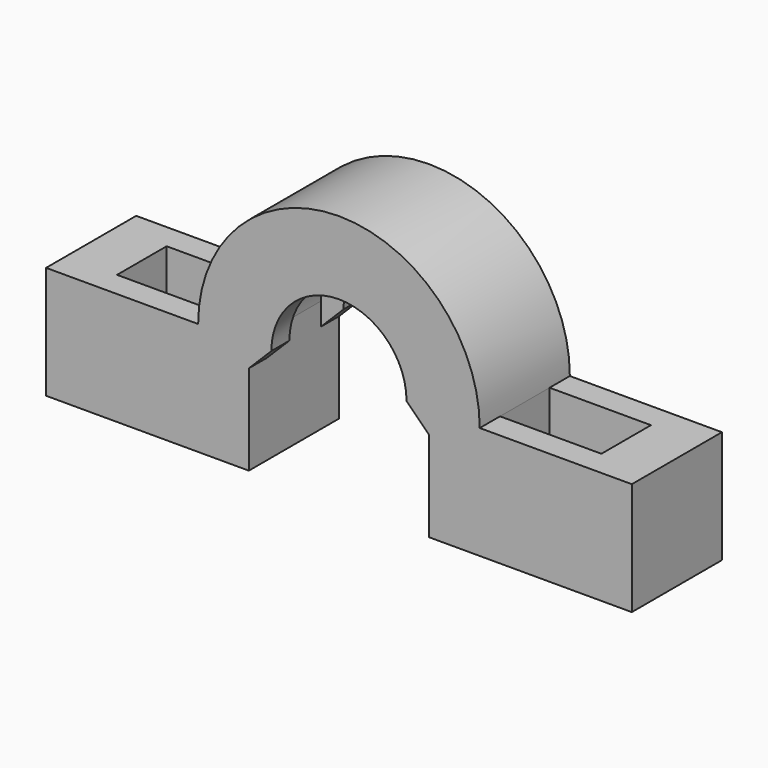
from build123d import *

# Parameters (mm, degrees)
F1_DEPTH      = 5
F1_DEPTH_BACK = 5
F3_DEPTH      = 2
F5_W          = 9
F5_H          = 5.5
F6_DEPTH      = 25
F7_SIZE       = 1.99999


# Not quite as in the source:
# - a fillet or chamfer is up to 0.001 mm smaller than in the source, because OpenCascade refuses the exact size


with BuildPart() as f1:
    # F0 (on Front) → F1 (new body, two sides)
    with BuildSketch(Plane.XZ) as f1_sk:
        with BuildLine():
            Line((8, 0), (12.5, 0))
            ThreePointArc((12.5, 0), (0, 12.5), (-12.5, 0))
            Line((-12.5, 0), (-8, 0))
            ThreePointArc((-8, 0), (0, 8), (8, 0))
        make_face()
        Polygon((26, 0), (12.5, 0), (8, 0), (8, -10), (26, -10), align=None)
        Polygon((-8, 0), (-12.5, 0), (-26, 0), (-26, -10), (-8, -10), align=None)
    extrude(amount=F1_DEPTH)
    extrude(f1_sk.sketch, amount=-F1_DEPTH_BACK)

    # F2 (on face) → F3 (join)
    with BuildSketch(Plane(origin=(0, 5, 0), x_dir=(-1, 0, 0), z_dir=(0, 1, 0))):
        with BuildLine():
            Line((6, 0), (8, 0))
            ThreePointArc((8, 0), (0, 8), (-8, 0))
            Line((-8, 0), (-6, 0))
            ThreePointArc((-6, 0), (0, 6), (6, 0))
        make_face()
    extrude(amount=-F3_DEPTH)

    # F4: F1 across plane


with BuildPart() as f1_1:
    add(f1.part)
    add(f1.part.mirror(Plane.XZ))

    # F5 (on face) → F6 (cut)
    with BuildSketch(Plane.XY):
        with Locations((-17, 0)):
            Rectangle(F5_W, F5_H)
        with Locations((17, 0)):
            Rectangle(F5_W, F5_H)
    extrude(amount=-F6_DEPTH, mode=Mode.SUBTRACT)

    # F7 (size 2 in the source; OpenCascade refuses exactly that, so slightly less here)
    f7_edges = [f1_1.edges().sort_by_distance(p)[0] for p in [
        (-8, -4, 0),
        (-8, 0, 0),
        (-8, 4, 0),
        (8, 0, 0),
        (8, -4, 0),
        (8, 4, 0),
    ]]
    chamfer(f7_edges, length=F7_SIZE)


solid = f1_1.part
